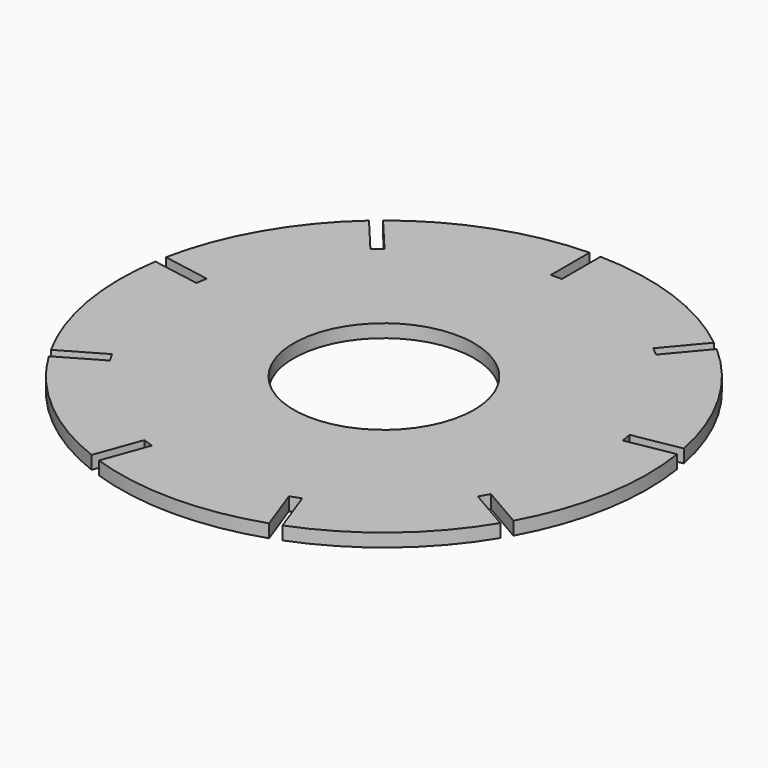
from build123d import *

# Parameters (mm, degrees)
F0_R            = 60
F0_R_2          = 20.5
F1_DEPTH        = 3
F2_W            = 2.5
F2_H            = 11
F3_DEPTH        = 25
F3_COPIES_COUNT = 9


# Not quite as in the source:
# - a pattern or mirror of a feature is missing from the dataset's text; its kind, count and spacing are read off the source's solid


with BuildPart() as f1:
    # F0 (on Top) → F1 (new body)
    with BuildSketch(Plane.XY):
        Circle(F0_R)
        Circle(F0_R_2, mode=Mode.SUBTRACT)
    extrude(amount=F1_DEPTH)

    # F2 (on Top) → F3 (cut)
    with BuildSketch(Plane.XY):
        with Locations((0, 54.5)):
            Rectangle(F2_W, F2_H)
    f3 = extrude(amount=F3_DEPTH, mode=Mode.SUBTRACT)

    # F3_copies: F3 ×9 about axis
    f3_copies_axis = Axis((0, 0, 0), (0, 0, 1))
    for i in range(1, F3_COPIES_COUNT):
        add(f3.rotate(f3_copies_axis, i * 360 / F3_COPIES_COUNT), mode=Mode.SUBTRACT)


solid = f1.part
